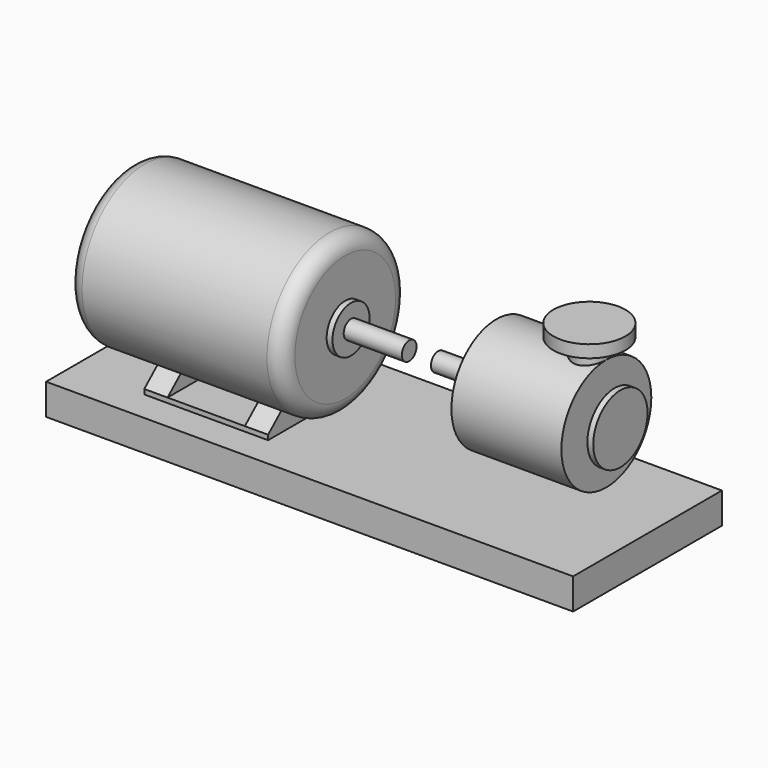
from build123d import *

# Parameters (mm, degrees)
F0_W     = 190.5
F0_H     = 30.1625
F2_DEPTH = 203.2
F4_DEPTH = 76.2
F6_DEPTH = 76.2
F7_DEPTH = 304.8
F0_W_2   = 26.924
F0_H_2   = 50.8
F0_W_3   = 55.626
F0_H_3   = 47.498
F0_H_4   = 184.15


with BuildPart() as f1:
    # F0 (on Front) → F1 (revolve)
    with BuildSketch(Plane.XZ):
        with BuildLine():
            ThreePointArc((-831.85, 117.4010858536), (-817.9268261091, 82.4620003458), (-783.7893820427, 66.675))
            Line((-783.7893820427, 66.675), (-623.0849027634, 66.675))
            Line((-623.0849027634, 66.675), (-234.2933673859, 66.675))
            Line((-234.2933673859, 66.675), (-234.2933673859, 323.85))
            Line((-234.2933673859, 323.85), (-831.85, 323.85))
            Line((-831.85, 323.85), (-831.85, 117.4010858536))
        make_face()
        with BuildLine():
            Line((-234.2933673859, 323.85), (-234.2933673859, 66.675))
            Line((-234.2933673859, 66.675), (-217.2845751047, 66.675))
            Line((-217.2845751047, 66.675), (-177.8, 66.675))
            ThreePointArc((-177.8, 66.675), (-141.8789755157, 81.5539755157), (-127, 117.475))
            Line((-127, 117.475), (-127, 247.65))
            Line((-127, 247.65), (-127, 323.85))
            Line((-127, 323.85), (-234.2933673859, 323.85))
        make_face()
        Polygon((-107.95, 323.85), (-127, 323.85), (-127, 247.65), (-107.95, 247.65), (-107.95, 293.6875), align=None)
        with Locations((-12.7, 308.76875)):
            Rectangle(F0_W, F0_H)
    revolve(axis=Axis((-374.65, 0, 323.85), (-1, 0, 0)))


with BuildPart() as f2:
    # F0 (on Front) → F2 (new body, symmetric)
    with BuildSketch(Plane.XZ):
        Polygon((-623.0849027634, 66.675), (-623.0849027634, 50.8), (-533.4, 50.8), (-217.2845751047, 50.8), (-217.2845751047, 66.675), (-234.2933673859, 66.675), align=None)
    extrude(amount=F2_DEPTH, both=True)

    # F3 (on face) → F4 (join)
    with BuildSketch(Plane(origin=(-623.0849027634, 0, 0), x_dir=(0, -1, 0), z_dir=(-1, 0, 0))):
        Polygon((0, 244.475), (0, 66.675), (203.2, 66.675), align=None)
        Polygon((-203.2, 66.675), (0, 66.675), (0, 244.475), align=None)
    extrude(amount=-F4_DEPTH)

    # F5 (on face) → F6 (join)
    with BuildSketch(Plane.YZ.offset(-217.2845751047)):
        Polygon((-203.2, 66.675), (0, 66.675), (0, 244.475), align=None)
        Polygon((0, 244.475), (0, 66.675), (203.2, 66.675), align=None)
    extrude(amount=-F6_DEPTH)

    # F0 (on Front) → F7 (join, symmetric)
    with BuildSketch(Plane.XZ):
        Polygon((-863.6, 50.8), (-863.6, -50.8), (863.6, -50.8), (863.6, 50.8), (705.2845358849, 50.8), (588.1003141403, 50.8), (455.1412463188, 50.8), (368.3, 50.8), (-127, 50.8), (-217.2845751047, 50.8), (-533.4, 50.8), (-623.0849027634, 50.8), (-736.6, 50.8), (-831.85, 50.8), align=None)
    extrude(amount=F7_DEPTH, both=True)


with BuildPart() as f8:
    # F0 (on Front) → F8 (revolve)
    with BuildSketch(Plane.XZ):
        with Locations((273.05, 308.76875)):
            Rectangle(F0_W, F0_H)
        Polygon((615.1428222656, 139.7), (689.5097494125, 139.7), (728.726, 139.7), (728.726, 273.05), (728.726, 323.85), (673.1, 323.85), (617.474, 323.85), (368.3, 323.85), (368.3, 293.6875), (368.3, 139.7), (394.2955732346, 139.7), (455.1412463188, 139.7), align=None)
        with Locations((742.188, 298.45)):
            Rectangle(F0_W_2, F0_H_2)
        Polygon((755.65, 323.85), (755.65, 273.05), (755.65, 212.598), (774.7, 212.598), (774.7, 323.85), align=None)
    revolve(axis=Axis((476.25, 0, 323.85), (-1, 0, 0)))

    # F0 (on Front) → F9 (revolve)
    with BuildSketch(Plane.XZ):
        Polygon((617.474, 555.498), (673.1, 555.498), (673.1, 596.0371494293), (555.0411343575, 596.0371494293), (555.0411343575, 555.498), align=None)
        with Locations((645.287, 531.749)):
            Rectangle(F0_W_3, F0_H_3)
        with Locations((645.287, 415.925)):
            Rectangle(F0_W_3, F0_H_4)
    revolve(axis=Axis((673.1, 0, 439.674), (0, 0, -1)))


solid = Compound([f1.part, f2.part, f8.part])
